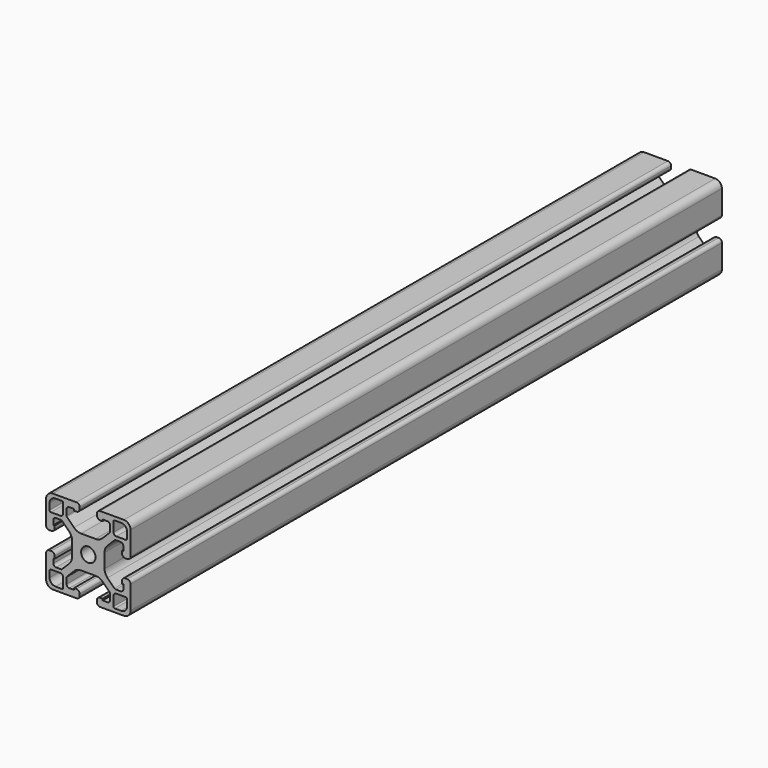
from build123d import *

# Parameters (mm, degrees)
F0_R     = 3.4
F1_DEPTH = 350


# Not quite as in the source:
# - ends of sketch curves that miss each other by under 0.0002 mm in the source are joined


with BuildPart() as f1:
    # F0 (on Front) → F1 (new body)
    with BuildSketch(Plane.XZ):
        with BuildLine():
            ThreePointArc((9.0741494418, -6.7149045575), (8.0460058013, -5.1746202437), (7.685, -3.358242))
            Line((7.685, -3.358242), (7.685, 3.358242))
            ThreePointArc((7.685, 3.358242), (8.0460058013, 5.1746202437), (9.0741494418, 6.7149045575))
            Line((9.0741494418, 6.7149045575), (12.373455, 10.018326))
            ThreePointArc((12.373455, 10.018326), (12.6623276754, 10.2115396696), (13.003172, 10.279393))
            Line((13.003172, 10.279393), (15.29885, 10.279393))
            ThreePointArc((15.29885, 10.279393), (16.1968756121, 9.9074186121), (16.56885, 9.009393))
            Line((16.56885, 9.009393), (16.56885, 6.901426))
            Line((16.56885, 6.901426), (15.94, 6.901426))
            Line((15.94, 6.901426), (15.94, 5.758104))
            ThreePointArc((15.94, 5.758104), (16.3998423535, 4.6479463535), (17.51, 4.188104))
            Line((17.51, 4.188104), (18.43, 4.188104))
            ThreePointArc((18.43, 4.188104), (19.5401576465, 4.6479463535), (20, 5.758104))
            Line((20, 5.758104), (20, 16.83))
            ThreePointArc((20, 16.83), (19.0715284964, 19.0715284964), (16.83, 20))
            Line((16.83, 20), (5.63, 20))
            ThreePointArc((5.63, 20), (4.5198423535, 19.5401576465), (4.06, 18.43))
            Line((4.06, 18.43), (4.06, 17.696221))
            ThreePointArc((4.06, 17.696221), (4.5198423535, 16.5860633535), (5.63, 16.126221))
            Line((5.63, 16.126221), (6.783928, 16.126221))
            Line((6.783928, 16.126221), (6.783928, 16.886684))
            Line((6.783928, 16.886684), (9.015, 16.886684))
            ThreePointArc((9.015, 16.886684), (9.9130256121, 16.5147096121), (10.285, 15.616684))
            Line((10.285, 15.616684), (10.285, 12.922194))
            ThreePointArc((10.285, 12.922194), (10.2548511553, 12.6925072769), (10.1664472118, 12.4783818782))
            Line((10.1664472118, 12.4783818782), (6.770639, 9.078337))
            ThreePointArc((6.770639, 9.078337), (5.2289028603, 8.0471389307), (3.409789, 7.685))
            Line((3.409789, 7.685), (-3.409789, 7.685))
            ThreePointArc((-3.409789, 7.685), (-5.2289028603, 8.0471389307), (-6.7706390582, 9.0783369418))
            Line((-6.7706390582, 9.0783369418), (-10.166447, 12.478382))
            ThreePointArc((-10.166447, 12.478382), (-10.2548511553, 12.6925072769), (-10.285, 12.922194))
            Line((-10.285, 12.922194), (-10.285, 15.616684))
            ThreePointArc((-10.285, 15.616684), (-9.9130256121, 16.5147096121), (-9.015, 16.886684))
            Line((-9.015, 16.886684), (-6.783928, 16.886684))
            Line((-6.783928, 16.886684), (-6.783928, 16.126221))
            Line((-6.783928, 16.126221), (-5.63, 16.126221))
            ThreePointArc((-5.63, 16.126221), (-4.5198423535, 16.5860633535), (-4.06, 17.696221))
            Line((-4.06, 17.696221), (-4.06, 18.43))
            ThreePointArc((-4.06, 18.43), (-4.5198423535, 19.5401576465), (-5.63, 20))
            Line((-5.63, 20), (-16.83, 20))
            ThreePointArc((-16.83, 20), (-19.0715284964, 19.0715284964), (-20, 16.83))
            Line((-20, 16.83), (-20, 5.758104))
            ThreePointArc((-20, 5.758104), (-19.5401576465, 4.6479463535), (-18.43, 4.188104))
            Line((-18.43, 4.188104), (-17.51, 4.188104))
            ThreePointArc((-17.51, 4.188104), (-16.3998423535, 4.6479463535), (-15.94, 5.758104))
            Line((-15.94, 5.758104), (-15.94, 6.901426))
            Line((-15.94, 6.901426), (-16.56885, 6.901426))
            Line((-16.56885, 6.901426), (-16.56885, 9.009393))
            ThreePointArc((-16.56885, 9.009393), (-16.1968756121, 9.9074186121), (-15.29885, 10.279393))
            Line((-15.29885, 10.279393), (-13.003172, 10.279393))
            ThreePointArc((-13.003172, 10.279393), (-12.6623276754, 10.2115396696), (-12.3734550869, 10.0183259132))
            Line((-12.3734550869, 10.0183259132), (-9.07415, 6.714904))
            ThreePointArc((-9.07415, 6.714904), (-8.0460058013, 5.1746202437), (-7.685, 3.358242))
            Line((-7.685, 3.358242), (-7.685, -3.358242))
            ThreePointArc((-7.685, -3.358242), (-8.0460058013, -5.1746202437), (-9.0741494418, -6.7149045575))
            Line((-9.0741494418, -6.7149045575), (-12.373455, -10.018326))
            ThreePointArc((-12.373455, -10.018326), (-12.6623276754, -10.2115396696), (-13.003172, -10.279393))
            Line((-13.003172, -10.279393), (-15.29885, -10.279393))
            ThreePointArc((-15.29885, -10.279393), (-16.1968756121, -9.9074186121), (-16.56885, -9.009393))
            Line((-16.56885, -9.009393), (-16.56885, -6.901426))
            Line((-16.56885, -6.901426), (-15.94, -6.901426))
            Line((-15.94, -6.901426), (-15.94, -5.758104))
            ThreePointArc((-15.94, -5.758104), (-16.3998423535, -4.6479463535), (-17.51, -4.188104))
            Line((-17.51, -4.188104), (-18.43, -4.188104))
            ThreePointArc((-18.43, -4.188104), (-19.5401576465, -4.6479463535), (-20, -5.758104))
            Line((-20, -5.758104), (-20, -16.83))
            ThreePointArc((-20, -16.83), (-19.0715284964, -19.0715284964), (-16.83, -20))
            Line((-16.83, -20), (-5.63, -20))
            ThreePointArc((-5.63, -20), (-4.5198423535, -19.5401576465), (-4.06, -18.43))
            Line((-4.06, -18.43), (-4.06, -17.696221))
            ThreePointArc((-4.06, -17.696221), (-4.5198423535, -16.5860633535), (-5.63, -16.126221))
            Line((-5.63, -16.126221), (-6.783928, -16.126221))
            Line((-6.783928, -16.126221), (-6.783928, -16.886684))
            Line((-6.783928, -16.886684), (-9.015, -16.886684))
            ThreePointArc((-9.015, -16.886684), (-9.9130256121, -16.5147096121), (-10.285, -15.616684))
            Line((-10.285, -15.616684), (-10.285, -12.922194))
            ThreePointArc((-10.285, -12.922194), (-10.2548511553, -12.6925072769), (-10.1664472118, -12.4783818782))
            Line((-10.1664472118, -12.4783818782), (-6.770639, -9.078337))
            ThreePointArc((-6.770639, -9.078337), (-5.2289028603, -8.0471389307), (-3.409789, -7.685))
            Line((-3.409789, -7.685), (3.409789, -7.685))
            ThreePointArc((3.409789, -7.685), (5.2289028603, -8.0471389307), (6.7706390582, -9.0783369418))
            Line((6.7706390582, -9.0783369418), (10.166447, -12.478382))
            ThreePointArc((10.166447, -12.478382), (10.2548511553, -12.6925072769), (10.285, -12.922194))
            Line((10.285, -12.922194), (10.285, -15.616684))
            ThreePointArc((10.285, -15.616684), (9.9130256121, -16.5147096121), (9.015, -16.886684))
            Line((9.015, -16.886684), (6.783928, -16.886684))
            Line((6.783928, -16.886684), (6.783928, -16.126221))
            Line((6.783928, -16.126221), (5.63, -16.126221))
            ThreePointArc((5.63, -16.126221), (4.5198423535, -16.5860633535), (4.06, -17.696221))
            Line((4.06, -17.696221), (4.06, -18.43))
            ThreePointArc((4.06, -18.43), (4.5198423535, -19.5401576465), (5.63, -20))
            Line((5.63, -20), (16.83, -20))
            ThreePointArc((16.83, -20), (19.0715284964, -19.0715284964), (20, -16.83))
            Line((20, -16.83), (20, -5.758104))
            ThreePointArc((20, -5.758104), (19.5401576465, -4.6479463535), (18.43, -4.188104))
            Line((18.43, -4.188104), (17.51, -4.188104))
            ThreePointArc((17.51, -4.188104), (16.3998423535, -4.6479463535), (15.94, -5.758104))
            Line((15.94, -5.758104), (15.94, -6.901426))
            Line((15.94, -6.901426), (16.56885, -6.901426))
            Line((16.56885, -6.901426), (16.56885, -9.009393))
            ThreePointArc((16.56885, -9.009393), (16.1968756121, -9.9074186121), (15.29885, -10.279393))
            Line((15.29885, -10.279393), (13.003172, -10.279393))
            ThreePointArc((13.003172, -10.279393), (12.6623276754, -10.2115396696), (12.3734550869, -10.0183259132))
            Line((12.3734550869, -10.0183259132), (9.0741494418, -6.7149045575))
        make_face()
        with BuildLine():
            Line((-12.57, -18.35), (-15.55, -18.35))
            ThreePointArc((-15.55, -18.35), (-17.5298989873, -17.5298989873), (-18.35, -15.55))
            Line((-18.35, -15.55), (-18.35, -12.57))
            ThreePointArc((-18.35, -12.57), (-18.1654772721, -12.1245227279), (-17.72, -11.94))
            Line((-17.72, -11.94), (-13.21, -11.94))
            ThreePointArc((-13.21, -11.94), (-12.3119743879, -12.3119743879), (-11.94, -13.21))
            Line((-11.94, -13.21), (-11.94, -17.72))
            ThreePointArc((-11.94, -17.72), (-12.1245227279, -18.1654772721), (-12.57, -18.35))
        make_face(mode=Mode.SUBTRACT)
        with BuildLine():
            Line((13.21, -11.94), (17.72, -11.94))
            ThreePointArc((17.72, -11.94), (18.1654772721, -12.1245227279), (18.35, -12.57))
            Line((18.35, -12.57), (18.35, -15.55))
            ThreePointArc((18.35, -15.55), (17.5298989873, -17.5298989873), (15.55, -18.35))
            Line((15.55, -18.35), (12.57, -18.35))
            ThreePointArc((12.57, -18.35), (12.1245227279, -18.1654772721), (11.94, -17.72))
            Line((11.94, -17.72), (11.94, -13.21))
            ThreePointArc((11.94, -13.21), (12.3119743879, -12.3119743879), (13.21, -11.94))
        make_face(mode=Mode.SUBTRACT)
        with BuildLine():
            ThreePointArc((-17.72, 11.94), (-18.1654772721, 12.1245227279), (-18.35, 12.57))
            Line((-18.35, 12.57), (-18.35, 15.55))
            ThreePointArc((-18.35, 15.55), (-17.5298989873, 17.5298989873), (-15.55, 18.35))
            Line((-15.55, 18.35), (-12.57, 18.35))
            ThreePointArc((-12.57, 18.35), (-12.1245227279, 18.1654772721), (-11.94, 17.72))
            Line((-11.94, 17.72), (-11.94, 13.21))
            ThreePointArc((-11.94, 13.21), (-12.3119743879, 12.3119743879), (-13.21, 11.94))
            Line((-13.21, 11.94), (-17.72, 11.94))
        make_face(mode=Mode.SUBTRACT)
        Circle(F0_R, mode=Mode.SUBTRACT)
        with BuildLine():
            Line((12.57, 18.35), (15.55, 18.35))
            ThreePointArc((15.55, 18.35), (17.5298989873, 17.5298989873), (18.35, 15.55))
            Line((18.35, 15.55), (18.35, 12.57))
            ThreePointArc((18.35, 12.57), (18.1654772721, 12.1245227279), (17.72, 11.94))
            Line((17.72, 11.94), (13.21, 11.94))
            ThreePointArc((13.21, 11.94), (12.3119743879, 12.3119743879), (11.94, 13.21))
            Line((11.94, 13.21), (11.94, 17.72))
            ThreePointArc((11.94, 17.72), (12.1245227279, 18.1654772721), (12.57, 18.35))
        make_face(mode=Mode.SUBTRACT)
    extrude(amount=F1_DEPTH)


solid = f1.part
